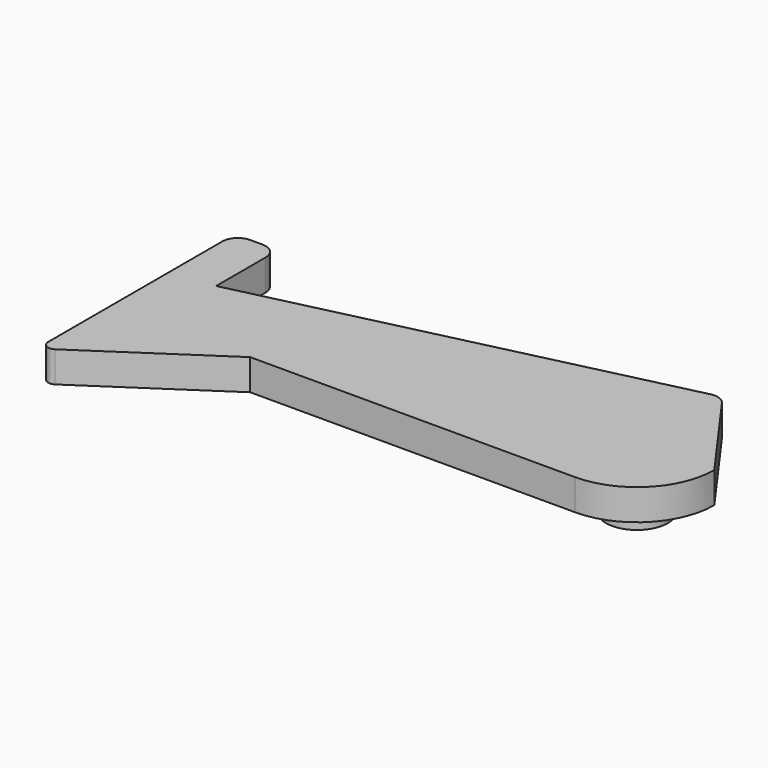
from build123d import *

# Parameters (mm, degrees)
F0_W     = 2.8
F0_H     = 5
F1_DEPTH = 2
F2_DEPTH = 2
F3_R     = 4.99999
F4_R     = 1
F5_R     = 1
F6_R     = 0.5


# Not quite as in the source:
# - a fillet or chamfer is up to 0.001 mm smaller than in the source, because OpenCascade refuses the exact size


with BuildPart() as f1:
    # F0 (on Top) → F1 (new body)
    with BuildSketch(Plane.XY):
        with BuildLine():
            Line((2.8, 0), (0, 0))
            Line((0, 0), (0, -5))
            Line((0, -5), (9, -5))
            Line((9, -5), (35, -5))
            Line((35, -5), (35, 0))
            Line((35, 0), (32, 0))
            ThreePointArc((32, 0), (30, -2), (28, 0))
            Line((28, 0), (2.8, 0))
        make_face()
        Polygon((9, -5), (0, -5), (0, -11), align=None)
        with BuildLine():
            Line((30.3363104735, 6.5), (2.8, 0))
            Line((2.8, 0), (28, 0))
            ThreePointArc((28, 0), (30, 2), (32, 0))
            Line((32, 0), (35, 0))
            Line((35, 0), (30.3363104735, 6.5))
        make_face()
        with Locations((1.4, 2.5)):
            Rectangle(F0_W, F0_H)
        with BuildLine():
            ThreePointArc((32, 0), (30, 2), (28, 0))
            Line((28, 0), (32, 0))
        make_face()
        with BuildLine():
            Line((32, 0), (28, 0))
            ThreePointArc((28, 0), (30, -2), (32, 0))
        make_face()
    extrude(amount=F1_DEPTH)

    # F3 (radius 5 in the source; OpenCascade refuses exactly that, so slightly less here)
    f3_edges = [f1.edges().sort_by_distance(p)[0] for p in [
        (35, -5, 1),
    ]]
    fillet(f3_edges, radius=F3_R)

    # F4
    f4_edges = [f1.edges().sort_by_distance(p)[0] for p in [
        (0, 5, 1),
        (2.8, 5, 1),
    ]]
    fillet(f4_edges, radius=F4_R)

    # F5
    f5_edges = [f1.edges().sort_by_distance(p)[0] for p in [
        (30.33631, 6.5, 1),
    ]]
    fillet(f5_edges, radius=F5_R)

    # F6
    f6_edges = [f1.edges().sort_by_distance(p)[0] for p in [
        (0, -11, 1),
    ]]
    fillet(f6_edges, radius=F6_R)


with BuildPart() as f2:
    # F0 (on Top) → F2 (new body)
    with BuildSketch(Plane.XY):
        with BuildLine():
            ThreePointArc((32, 0), (30, 2), (28, 0))
            Line((28, 0), (32, 0))
        make_face()
        with BuildLine():
            Line((32, 0), (28, 0))
            ThreePointArc((28, 0), (30, -2), (32, 0))
        make_face()
    extrude(amount=-F2_DEPTH)


solid = Compound([f1.part, f2.part])
